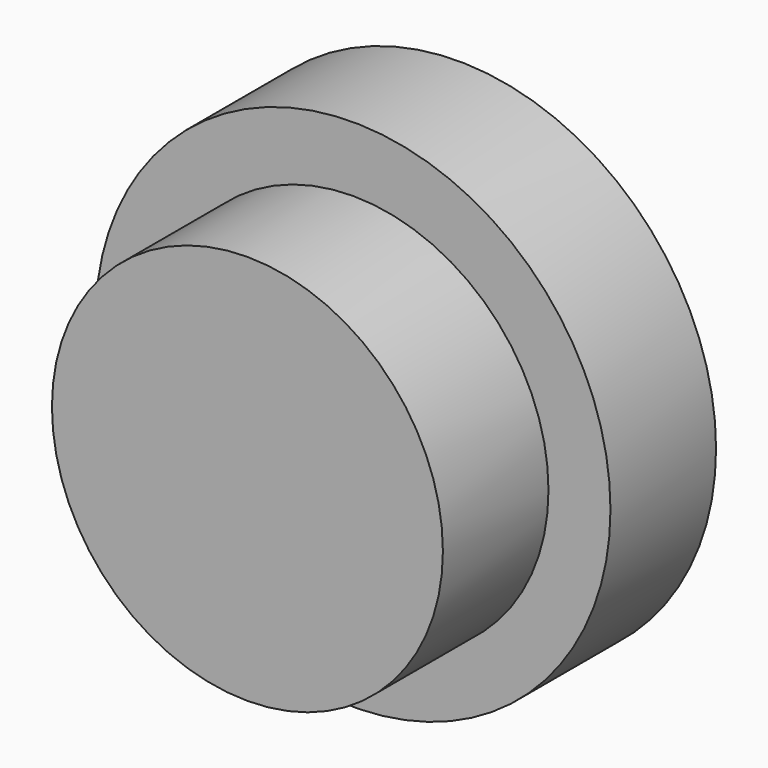
from build123d import *

# Parameters (mm, degrees)
F0_R     = 49.5467317532
F2_DEPTH = 25.4
F1_R     = 37.6187843243
F3_DEPTH = 25.4


with BuildPart() as f2:
    # F0 (on Front) → F2 (new body)
    with BuildSketch(Plane.XZ):
        with Locations((0, 22.9430384934)):
            Circle(F0_R)
    extrude(amount=F2_DEPTH)


with BuildPart() as f2b:
    # F1 (on face) → F2, piece 2 (new body)
    with BuildSketch(Plane.XZ):
        with Locations((0, 22.3517417908)):
            Circle(F1_R)
    extrude(amount=F2_DEPTH)


with BuildPart() as f3:
    # F3 (new): a face of the model
    f3_faces = [f2b.part.faces().sort_by_distance(p)[0] for p in [
        (0, -25.4, 22.3517417908),
    ]]
    extrude(f3_faces, amount=F3_DEPTH)


solid = Compound([f2.part, f2b.part, f3.part])
